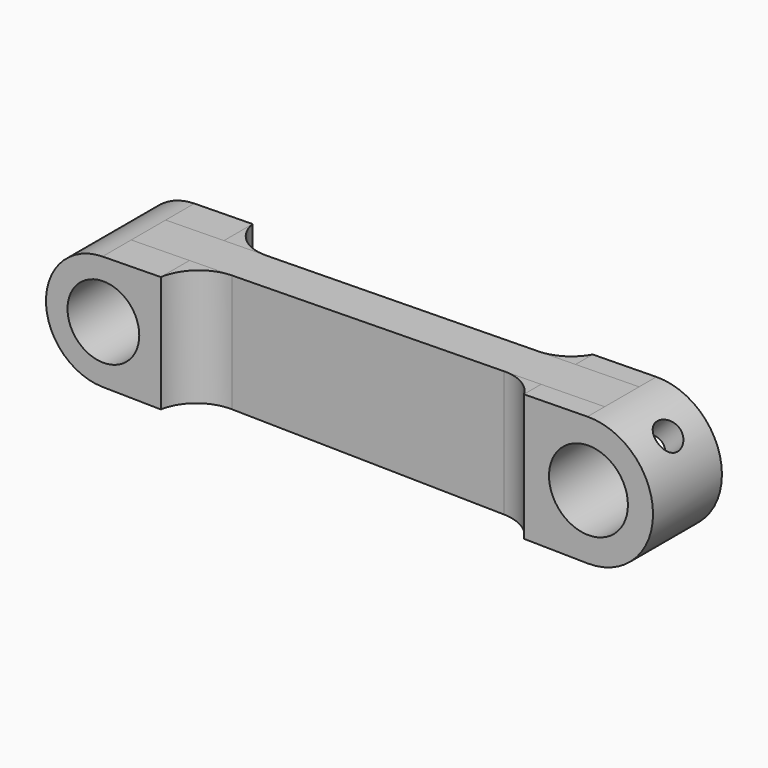
from build123d import *

# Parameters (mm, degrees)
F1_DEPTH      = 1.5
F1_DEPTH_BACK = 1.5
F3_DEPTH      = 4
F3_DEPTH_BACK = 4
F5_DEPTH      = 3
F5_DEPTH_BACK = 3
F6_R          = 2.5
F6_R_2        = 2.75
F7_DEPTH      = 4.001
F7_DEPTH_BACK = 4.001
F8_T4_DEPTH   = 22.9123439264
F8_T10_DEPTH  = 21.8550350011
F8_T16_DEPTH  = 21.8550350011
F8_T22_DEPTH  = 22.9123439264
F10_R         = 1
F11_DEPTH     = 6.3649610307


# Not quite as in the source:
# - a fillet or chamfer that OpenCascade refuses, or shapes differently, is made with other operations: its cross-section is extruded or revolved along the edge and cut away or added


with BuildPart() as f1:
    # F0 (on Front) → F1 (new body, two sides)
    with BuildSketch(Plane.XZ) as f1_sk:
        with BuildLine():
            Line((16.4318181818, 4.4994834414), (-16.5606060606, 3.9995408368))
            ThreePointArc((-16.5606060606, 3.9995408368), (-20.5, 0), (-16.5606060606, -3.9995408368))
            Line((-16.5606060606, -3.9995408368), (16.4318181818, -4.4994834414))
            ThreePointArc((16.4318181818, -4.4994834414), (21, 0), (16.4318181818, 4.4994834414))
        make_face()
    extrude(amount=F1_DEPTH)
    extrude(f1_sk.sketch, amount=-F1_DEPTH_BACK)

    # F2 (on Front) → F3 (join, two sides)
    with BuildSketch(Plane.XZ) as f3_sk:
        with BuildLine():
            Line((-12.5, 4.0610722343), (-16.5606060606, 3.9995408368))
            ThreePointArc((-16.5606060606, 3.9995408368), (-20.5, 0), (-16.5606060606, -3.9995408368))
            Line((-16.5606060606, -3.9995408368), (-12.5, -4.0610722343))
            Line((-12.5, -4.0610722343), (-12.5, 4.0610722343))
        make_face()
    extrude(amount=F3_DEPTH)
    extrude(f3_sk.sketch, amount=-F3_DEPTH_BACK)

    # F4 (on Front) → F5 (join, two sides)
    with BuildSketch(Plane.XZ) as f5_sk:
        with BuildLine():
            Line((16.4318181818, 4.4994834414), (12, 4.4323269722))
            Line((12, 4.4323269722), (12, -4.4323269722))
            Line((12, -4.4323269722), (16.4318181818, -4.4994834414))
            ThreePointArc((16.4318181818, -4.4994834414), (21, 0), (16.4318181818, 4.4994834414))
        make_face()
    extrude(amount=F5_DEPTH)
    extrude(f5_sk.sketch, amount=-F5_DEPTH_BACK)

    # F6 (on Front) → F7 (cut, two sides)
    with BuildSketch(Plane.XZ) as f7_sk:
        with Locations((-16.5, 0)):
            Circle(F6_R)
        with Locations((16.5, 0)):
            Circle(F6_R_2)
    extrude(amount=-F7_DEPTH, mode=Mode.SUBTRACT)
    extrude(f7_sk.sketch, amount=F7_DEPTH_BACK, mode=Mode.SUBTRACT)

    # F8: fillet of radius 3 on 4 edges, made by hand


with BuildPart() as f8_tool2:
    # F8_s3 → F8_t4 (new body)
    with BuildSketch(Plane.XY.offset(11.4561719632)):
        with BuildLine():
            ThreePointArc((-12.5, -4), (-11.4784517816, -2.2087121525), (-9.5419601084, -1.5))
            Line((-9.5419601084, -1.5), (-12.5, -1.5))
            Line((-12.5, -1.5), (-12.5, -4))
        make_face()
    extrude(amount=-F8_T4_DEPTH)

    split(bisect_by=Plane(origin=(-0.0643939394, 0, -4.2495121391), x_dir=(0, 1, 0), z_dir=(0.0151515152, 0, 0.9998852092)), keep=Keep.TOP)

    split(bisect_by=Plane(origin=(-0.0643939394, 0, 4.2495121391), x_dir=(0, 1, 0), z_dir=(0.0151515152, 0, -0.9998852092)), keep=Keep.TOP)


with BuildPart() as f1_1:
    add(f1.part)

    # F8_t1: union F8_tool2
    add(f8_tool2.part)


with BuildPart() as f8_tool8:
    # F8_s9 → F8_t10 (new body)
    with BuildSketch(Plane.XY.offset(-10.9275175005)):
        with BuildLine():
            ThreePointArc((9.4019237886, -1.5), (10.9019237886, -1.9019237886), (12, -3))
            Line((12, -3), (12, -1.5))
            Line((12, -1.5), (9.4019237886, -1.5))
        make_face()
    extrude(amount=F8_T10_DEPTH)

    split(bisect_by=Plane(origin=(-0.0643939394, 0, -4.2495121391), x_dir=(0, 1, 0), z_dir=(0.0151515152, 0, 0.9998852092)), keep=Keep.TOP)

    split(bisect_by=Plane(origin=(-0.0643939394, 0, 4.2495121391), x_dir=(0, 1, 0), z_dir=(0.0151515152, 0, -0.9998852092)), keep=Keep.TOP)


with BuildPart() as f1_2:
    add(f1_1.part)

    # F8_t7: union F8_tool8
    add(f8_tool8.part)


with BuildPart() as f8_tool14:
    # F8_s15 → F8_t16 (new body)
    with BuildSketch(Plane.XY.offset(-10.9275175005)):
        with BuildLine():
            ThreePointArc((12, 3), (10.9019237886, 1.9019237886), (9.4019237886, 1.5))
            Line((9.4019237886, 1.5), (12, 1.5))
            Line((12, 1.5), (12, 3))
        make_face()
    extrude(amount=F8_T16_DEPTH)

    split(bisect_by=Plane(origin=(-0.0643939394, 0, -4.2495121391), x_dir=(0, 1, 0), z_dir=(0.0151515152, 0, 0.9998852092)), keep=Keep.TOP)

    split(bisect_by=Plane(origin=(-0.0643939394, 0, 4.2495121391), x_dir=(0, 1, 0), z_dir=(0.0151515152, 0, -0.9998852092)), keep=Keep.TOP)


with BuildPart() as f1_3:
    add(f1_2.part)

    # F8_t13: union F8_tool14
    add(f8_tool14.part)


with BuildPart() as f8_tool20:
    # F8_s21 → F8_t22 (new body)
    with BuildSketch(Plane.XY.offset(11.4561719632)):
        with BuildLine():
            ThreePointArc((-9.5419601084, 1.5), (-11.4784517816, 2.2087121525), (-12.5, 4))
            Line((-12.5, 4), (-12.5, 1.5))
            Line((-12.5, 1.5), (-9.5419601084, 1.5))
        make_face()
    extrude(amount=-F8_T22_DEPTH)

    split(bisect_by=Plane(origin=(-0.0643939394, 0, -4.2495121391), x_dir=(0, 1, 0), z_dir=(0.0151515152, 0, 0.9998852092)), keep=Keep.TOP)

    split(bisect_by=Plane(origin=(-0.0643939394, 0, 4.2495121391), x_dir=(0, 1, 0), z_dir=(0.0151515152, 0, -0.9998852092)), keep=Keep.TOP)


with BuildPart() as f1_4:
    add(f1_3.part)

    # F8_t19: union F8_tool20
    add(f8_tool20.part)

    # F10 (on face) → F11 (cut, through all)
    with BuildSketch(Plane(origin=(8.25, 0, 8.25), x_dir=(0.7071067812, 0, -0.7071067812), z_dir=(0.7071067812, 0, 0.7071067812))):
        with Locations((11.6672618896, 0)):
            Circle(F10_R)
    extrude(amount=F11_DEPTH, mode=Mode.SUBTRACT)


solid = f1_4.part
